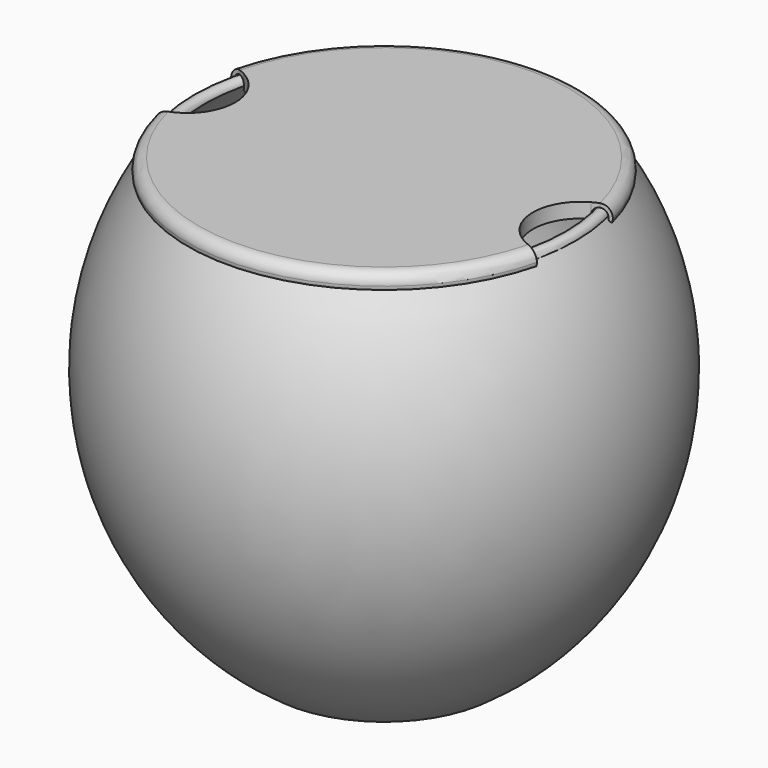
from build123d import *

# Parameters (mm, degrees)
F3_DEPTH = 25
F4_DEPTH = 3.005
F5_R     = 2.80499


# Not quite as in the source:
# - a fillet or chamfer is up to 0.001 mm smaller than in the source, because OpenCascade refuses the exact size


with BuildPart() as f1:
    # F0 (on Front) → F1 (revolve)
    with BuildSketch(Plane.XZ):
        with BuildLine():
            ThreePointArc((-39.3, 0), (-37.83, 1.47), (-36.36, 0))
            Line((-36.36, 0), (-35.56, 0))
            ThreePointArc((-35.56, 0), (-35.923724, 1.232481), (-36.898335, 2.07))
            ThreePointArc((-36.898335, 2.07), (-37.353555, 2.219437), (-37.83, 2.27))
            ThreePointArc((-37.83, 2.27), (-39.435132, 1.605132), (-40.1, 0))
            Line((-40.1, 0), (-39.3, 0))
        make_face()
        with BuildLine():
            ThreePointArc((-37.83, 2.27), (-37.353555, 2.219437), (-36.898335, 2.07))
            Line((-36.898335, 2.07), (-35.56, 2.07))
            Line((-35.56, 2.07), (0, 2.07))
            Line((0, 2.07), (0, 2.27))
            Line((0, 2.27), (-37.83, 2.27))
        make_face()
        with BuildLine():
            ThreePointArc((-36.898335, 2.07), (-35.923724, 1.232481), (-35.56, 0))
            Line((-35.56, 0), (-35.56, 2.07))
            Line((-35.56, 2.07), (-36.898335, 2.07))
        make_face()
        with BuildLine():
            ThreePointArc((-39.103057, -0.735), (-39.249911, -0.380464), (-39.3, 0))
            Line((-39.3, 0), (-40.1, 0))
            ThreePointArc((-40.1, 0), (-40.06922, -0.372552), (-39.977714, -0.735))
            Line((-39.977714, -0.735), (-39.103057, -0.735))
        make_face()
        with BuildLine():
            Line((-35.56, 0), (-36.36, 0))
            ThreePointArc((-36.36, 0), (-36.410089, -0.380464), (-36.556943, -0.735))
            Line((-36.556943, -0.735), (-35.682286, -0.735))
            ThreePointArc((-35.682286, -0.735), (-35.59078, -0.372552), (-35.56, 0))
        make_face()
        with BuildLine():
            Line((-35.56, -0.735), (-35.56, 0))
            ThreePointArc((-35.56, 0), (-35.59078, -0.372552), (-35.682286, -0.735))
            Line((-35.682286, -0.735), (-35.56, -0.735))
        make_face()
    revolve(axis=Axis((0, 0, 2.17), (0, 0, 1)))

    # F2 (on face) → F3 (cut)
    with BuildSketch(Plane.XY.offset(2.27)):
        with BuildLine():
            ThreePointArc((36.708933, -9.141289), (45.667746, -8.003918), (49.85, 0))
            ThreePointArc((49.85, 0), (45.667746, 8.003918), (36.708933, 9.141289))
            ThreePointArc((36.708933, 9.141289), (37.548687, 4.604887), (37.83, 0))
            ThreePointArc((37.83, 0), (37.548687, -4.604887), (36.708933, -9.141289))
        make_face()
        with BuildLine():
            ThreePointArc((37.83, 0), (37.548687, 4.604887), (36.708933, 9.141289))
            ThreePointArc((36.708933, 9.141289), (36.016955, 8.853883), (35.349091, 8.514186))
            ThreePointArc((35.349091, 8.514186), (36.106388, 4.286995), (36.36, 0))
            ThreePointArc((36.36, 0), (36.106388, -4.286995), (35.349091, -8.514186))
            ThreePointArc((35.349091, -8.514186), (36.016955, -8.853883), (36.708933, -9.141289))
            ThreePointArc((36.708933, -9.141289), (37.548687, -4.604887), (37.83, 0))
        make_face()
        with BuildLine():
            ThreePointArc((-35.349091, 8.514186), (-36.016955, 8.853883), (-36.708933, 9.141289))
            ThreePointArc((-36.708933, 9.141289), (-37.83, 0), (-36.708933, -9.141289))
            ThreePointArc((-36.708933, -9.141289), (-36.016955, -8.853883), (-35.349091, -8.514186))
            ThreePointArc((-35.349091, -8.514186), (-36.36, 0), (-35.349091, 8.514186))
        make_face()
        with BuildLine():
            ThreePointArc((-36.708933, -9.141289), (-37.83, 0), (-36.708933, 9.141289))
            ThreePointArc((-36.708933, 9.141289), (-49.85, 0), (-36.708933, -9.141289))
        make_face()
        with BuildLine():
            ThreePointArc((36.36, 0), (36.106388, 4.286995), (35.349091, 8.514186))
            ThreePointArc((35.349091, 8.514186), (30.35, 0), (35.349091, -8.514186))
            ThreePointArc((35.349091, -8.514186), (36.106388, -4.286995), (36.36, 0))
        make_face()
        with BuildLine():
            ThreePointArc((-30.35, 0), (-31.692151, 4.936656), (-35.349091, 8.514186))
            ThreePointArc((-35.349091, 8.514186), (-36.36, 0), (-35.349091, -8.514186))
            ThreePointArc((-35.349091, -8.514186), (-31.692151, -4.936656), (-30.35, 0))
        make_face()
    extrude(amount=-F3_DEPTH, mode=Mode.SUBTRACT)

    # F2 (on face) → F4 (join, through all)
    with BuildSketch(Plane.XY.offset(2.27)):
        with BuildLine():
            ThreePointArc((35.349091, -8.514186), (30.35, 0), (35.349091, 8.514186))
            ThreePointArc((35.349091, 8.514186), (35.250117, 8.915089), (35.146597, 9.314843))
            ThreePointArc((35.146597, 9.314843), (29.55, 0), (35.146597, -9.314843))
            ThreePointArc((35.146597, -9.314843), (35.250117, -8.915089), (35.349091, -8.514186))
        make_face()
        with BuildLine():
            ThreePointArc((-29.55, 0), (-31.056746, 5.43342), (-35.146597, 9.314843))
            ThreePointArc((-35.146597, 9.314843), (-35.250117, 8.915089), (-35.349091, 8.514186))
            ThreePointArc((-35.349091, 8.514186), (-31.692151, 4.936656), (-30.35, 0))
            ThreePointArc((-30.35, 0), (-31.692151, -4.936656), (-35.349091, -8.514186))
            ThreePointArc((-35.349091, -8.514186), (-35.250117, -8.915089), (-35.146597, -9.314843))
            ThreePointArc((-35.146597, -9.314843), (-31.056746, -5.43342), (-29.55, 0))
        make_face()
    extrude(amount=-F4_DEPTH)

    # F5 (radius 2.805 in the source; OpenCascade refuses exactly that, so slightly less here)
    f5_edges = [f1.edges().sort_by_distance(p)[0] for p in [
        (-29.55, 0, 2.07),
        (0, 35.56, 2.07),
        (29.55, 0, 2.07),
        (0, -35.56, 2.07),
    ]]
    fillet(f5_edges, radius=F5_R)


with BuildPart() as f7:
    # F6 (on Front) → F7 (revolve)
    with BuildSketch(Plane.XZ):
        with BuildLine():
            ThreePointArc((-23.097345, -84.515505), (-47.332407, -45.045959), (-36.56, 0))
            ThreePointArc((-36.56, 0), (-37.83, 1.27), (-39.1, 0))
            ThreePointArc((-39.1, 0), (-49.128458, -46.842011), (-23.097345, -87.055505))
            Line((-23.097345, -87.055505), (0, -87.055505))
            Line((0, -87.055505), (0, -84.515505))
            Line((0, -84.515505), (-23.097345, -84.515505))
        make_face()
    revolve(axis=Axis((0, 0, 2.17), (0, 0, 1)))


solid = Compound([f1.part, f7.part])
